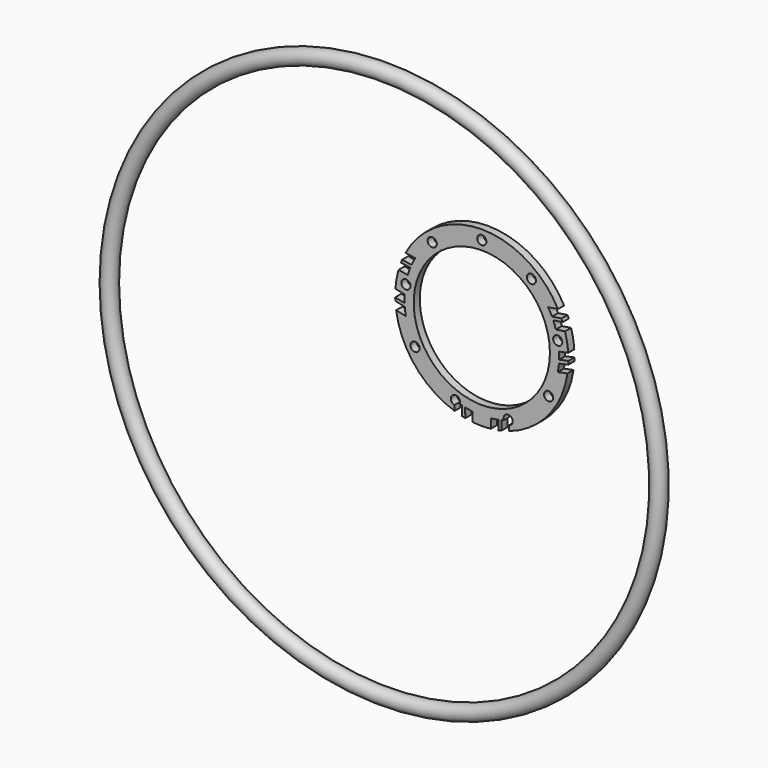
from build123d import *

# Parameters (mm, degrees)
F1_R     = 5
F3_START = -80
F0_R     = 3
F0_R_2   = 44.65
F3_DEPTH = 5


# Not quite as in the source:
# - the program builds the solid bodies; features that only make, move or delete a surface that nothing else refers to are left out


with BuildPart() as f2:
    # F1 (on Top) → F2 (revolve)
    with BuildSketch(Plane.XY):
        with Locations((-180.1196336746, 0)):
            Circle(F1_R)
    revolve(axis=Axis((0, 0, 0), (0, -1, 0)))


with BuildPart() as f3:
    # F0 (on Front) → F3 (new body)
    with BuildSketch(Plane.XZ.offset(F3_START)):
        with BuildLine():
            ThreePointArc((49.8109044328, -9.451568881), (50.0390468759, -8.1579496494), (50.2335990607, -6.8588541417))
            ThreePointArc((50.2335990607, -6.8588541417), (50.3944303881, -5.5551544159), (50.5214328951, -4.247725621))
            Line((50.5214328951, -4.247725621), (56.6710935634, -2.9915972871))
            ThreePointArc((56.6710935634, -2.9915972871), (56.7192812989, -1.8669839158), (56.7451537669, -0.7416360104))
            Line((56.7451537669, -0.7416360104), (50.6608373732, -1.9844171372))
            ThreePointArc((50.6608373732, -1.9844171372), (50.6930409681, -0.8209458797), (50.6985279324, 0.342958039))
            ThreePointArc((50.6985279324, 0.342958039), (50.6772953744, 1.5066812093), (50.6293544842, 2.669610317))
            Line((50.6293544842, 2.669610317), (56.6163478884, 3.8925122714))
            ThreePointArc((56.6163478884, 3.8925122714), (55.8979189272, 9.7972016216), (54.5653885403, 15.5942577074))
            Line((54.5653885403, 15.5942577074), (48.5235922547, 14.6941944125))
            ThreePointArc((48.5235922547, 14.6941944125), (48.1407923431, 15.9035363146), (47.7278574814, 17.1029229947))
            ThreePointArc((47.7278574814, 17.1029229947), (47.2850461567, 18.2916036663), (46.812635558, 19.4688342447))
            Line((46.812635558, 19.4688342447), (52.962392865, 20.384980795))
            ThreePointArc((52.962392865, 20.384980795), (52.5868512377, 21.3350785541), (52.1942673065, 22.2782620583))
            Line((52.1942673065, 22.2782620583), (45.9837474764, 21.353063545))
            ThreePointArc((45.9837474764, 21.353063545), (45.4151184326, 22.537199748), (44.8160027703, 23.7062070021))
            ThreePointArc((44.8160027703, 23.7062070021), (44.1868026685, 24.8593005667), (43.5279405017, 25.9957063842))
            Line((43.5279405017, 25.9957063842), (49.9419120736, 26.9512136727))
            ThreePointArc((49.9419120736, 26.9512136727), (-0.0180046804, 56.7499971439), (-49.9590032696, 26.9195187979))
            Line((-49.9590032696, 26.9195187979), (-43.5628595995, 25.9371474577))
            ThreePointArc((-43.5628595995, 25.9371474577), (-44.2201896339, 24.7998625696), (-44.847835498, 23.6459300066))
            ThreePointArc((-44.847835498, 23.6459300066), (-45.4453758651, 22.4761243815), (-46.0124096177, 21.2912309626))
            Line((-46.0124096177, 21.2912309626), (-52.2093042453, 22.2430000275))
            ThreePointArc((-52.2093042453, 22.2430000275), (-52.6107220584, 21.2761468431), (-52.9942367056, 20.3020534921))
            Line((-52.9942367056, 20.3020534921), (-46.8579202223, 19.3595885072))
            ThreePointArc((-46.8579202223, 19.3595885072), (-47.3185959, 18.2046377822), (-47.7508093952, 17.0387369495))
            ThreePointArc((-47.7508093952, 17.0387369495), (-48.154300731, 15.8625872996), (-48.5288272071, 14.6768962876))
            Line((-48.5288272071, 14.6768962876), (-54.5627095565, 15.6036286119))
            ThreePointArc((-54.5627095565, 15.6036286119), (-55.8869108783, 9.8598018482), (-56.6081759757, 4.0096025617))
            Line((-56.6081759757, 4.0096025617), (-50.6245477239, 2.7592612205))
            ThreePointArc((-50.6245477239, 2.7592612205), (-50.6769730719, 1.517483112), (-50.6989432189, 0.2747930459))
            ThreePointArc((-50.6989432189, 0.2747930459), (-50.6904449614, -0.9680621618), (-50.6514834065, -2.2103355958))
            Line((-50.6514834065, -2.2103355958), (-56.7422540571, -0.9376057363))
            ThreePointArc((-56.7422540571, -0.9376057363), (-56.7153067125, -1.9840575867), (-56.669062139, -3.029834367))
            Line((-56.669062139, -3.029834367), (-50.5156761211, -4.3156483586))
            ThreePointArc((-50.5156761211, -4.3156483586), (-50.3869158777, -5.6229052157), (-50.2243318582, -6.9263875238))
            ThreePointArc((-50.2243318582, -6.9263875238), (-50.0280332022, -8.2252202799), (-49.7981516812, -9.5185316024))
            Line((-49.7981516812, -9.5185316024), (-56.1559097911, -8.1900119371))
            ThreePointArc((-56.1559097911, -8.1900119371), (-43.4812708484, -36.4683641723), (-17.8413278177, -53.8725303072))
            Line((-17.8413278177, -53.8725303072), (-17.9232978779, -50.4336652809))
            ThreePointArc((-17.9232978779, -50.4336652809), (-19.1729257063, -45.1666666044), (-14.2891182451, -47.5014619807))
            ThreePointArc((-14.2891182451, -47.5014619807), (-14.3401340199, -48.0523630966), (-14.4914462714, -48.5845277809))
            ThreePointArc((-14.4914462714, -48.5845277809), (-13.7472884724, -48.8003116218), (-12.9999199783, -49.004698094))
            Line((-12.9999199783, -49.004698094), (-12.8504364982, -55.2759331157))
            ThreePointArc((-12.8504364982, -55.2759331157), (-11.8192358816, -55.5055687582), (-10.7839392307, -55.7159685788))
            Line((-10.7839392307, -55.7159685788), (-10.9319365624, -49.5070814907))
            ThreePointArc((-10.9319365624, -49.5070814907), (-9.7241474559, -49.7584094499), (-8.5106008637, -49.9802763865))
            ThreePointArc((-8.5106008637, -49.9802763865), (-7.2920153041, -50.1725509371), (-6.0691122787, -50.3351192596))
            Line((-6.0691122787, -50.3351192596), (-5.9235940949, -56.4399994064))
            ThreePointArc((-5.9235940949, -56.4399994064), (-0.0128386472, -56.7499985477), (5.8980564587, -56.4426738382))
            Line((5.8980564587, -56.4426738382), (6.0561074621, -50.3366855994))
            ThreePointArc((6.0561074621, -50.3366855994), (7.2855339368, -50.1734925034), (8.5106008637, -49.9802763865))
            ThreePointArc((8.5106008637, -49.9802763865), (9.7305751823, -49.7571528662), (10.9447268793, -49.5042554561))
            Line((10.9447268793, -49.5042554561), (10.7839392307, -55.7159685788))
            ThreePointArc((10.7839392307, -55.7159685788), (11.8127478396, -55.5069499115), (12.837513908, -55.278935741))
            Line((12.837513908, -55.278935741), (12.9999199783, -49.004698094))
            ThreePointArc((12.9999199783, -49.004698094), (13.7472884724, -48.8003116218), (14.4914462714, -48.5845277809))
            ThreePointArc((14.4914462714, -48.5845277809), (16.7382171293, -44.5524777555), (20.2891182451, -47.5014619807))
            ThreePointArc((20.2891182451, -47.5014619807), (19.6231430112, -49.3862241385), (17.9208993176, -50.434183017))
            Line((17.9208993176, -50.434183017), (17.831817606, -53.8756789365))
            ThreePointArc((17.831817606, -53.8756789365), (43.489586701, -36.4584468755), (56.1610799396, -8.1544834304))
            Line((56.1610799396, -8.1544834304), (49.8109044328, -9.451568881))
        make_face()
        with Locations((-43.7775841613, -25.275)):
            Circle(F0_R, mode=Mode.SUBTRACT)
        with Locations((43.7775841613, -25.275)):
            Circle(F0_R, mode=Mode.SUBTRACT)
        with Locations((-49.7820319148, 8.7779153811)):
            Circle(F0_R, mode=Mode.SUBTRACT)
        with Locations((-32.4929136697, 38.7235465997)):
            Circle(F0_R, mode=Mode.SUBTRACT)
        Circle(F0_R_2, mode=Mode.SUBTRACT)
        with Locations((32.4929136697, 38.7235465997)):
            Circle(F0_R, mode=Mode.SUBTRACT)
        with Locations((49.7820319148, 8.7779153811)):
            Circle(F0_R, mode=Mode.SUBTRACT)
        with Locations((0, 50.55)):
            Circle(F0_R, mode=Mode.SUBTRACT)
    extrude(amount=-F3_DEPTH)


solid = Compound([f2.part, f3.part])
